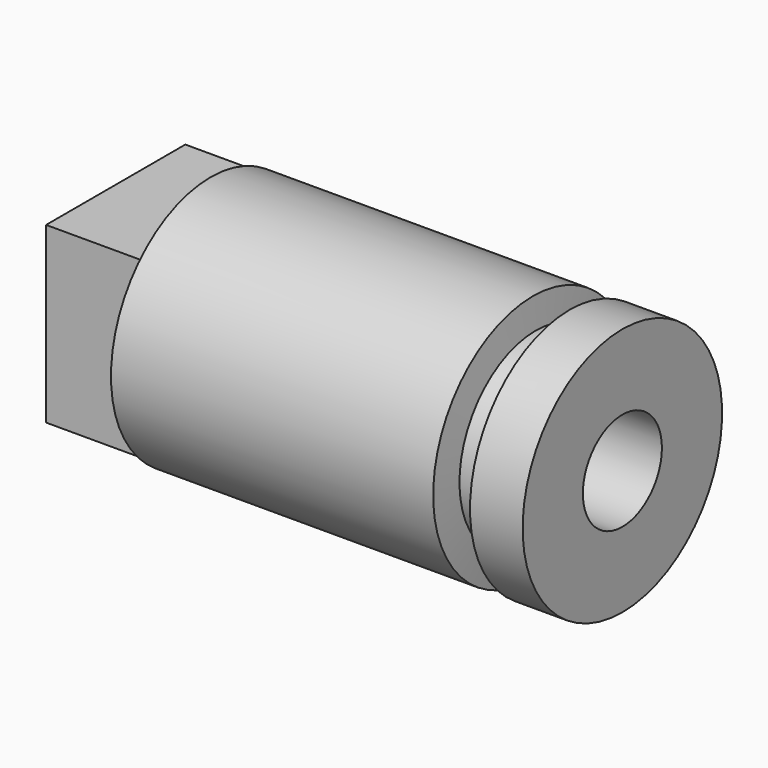
from build123d import *

# Parameters (mm, degrees)
F2_W     = 17.4498
F2_H     = 17.4498
F3_DEPTH = 9.525
F4_R     = 4.953
F5_DEPTH = 50.8


# Not quite as in the source:
# - a feature names something its author has since deleted; it is built from what else it names


with BuildPart() as f1:
    # F0 (on Front) → F1 (revolve)
    with BuildSketch(Plane.XZ):
        Polygon((-22.0124394905, 12.4968), (-22.0124394905, 7.5298989686), (-22.0124394905, 0), (19.2625605095, 0), (19.2625605095, 3.7935770415), (19.2625605095, 12.4968), (13.9844405095, 12.4968), (13.7253605095, 9.525), (10.5503605095, 9.525), (10.2912805095, 12.4968), align=None)
    revolve(axis=Axis((-1.3749394905, 0, 0), (1, 0, 0)))

    # F2 (on face) → F3 (join)
    with BuildSketch(Plane(origin=(-22.0124394905, 0, 0), x_dir=(0, -1, 0), z_dir=(-1, 0, 0))):
        Rectangle(F2_W, F2_H)
    extrude(amount=F3_DEPTH)

    # F4 (on face) → F5 (cut)
    with BuildSketch(Plane.YZ.offset(19.2625605095)):
        Circle(F4_R)
    extrude(amount=-F5_DEPTH, mode=Mode.SUBTRACT)


solid = f1.part
